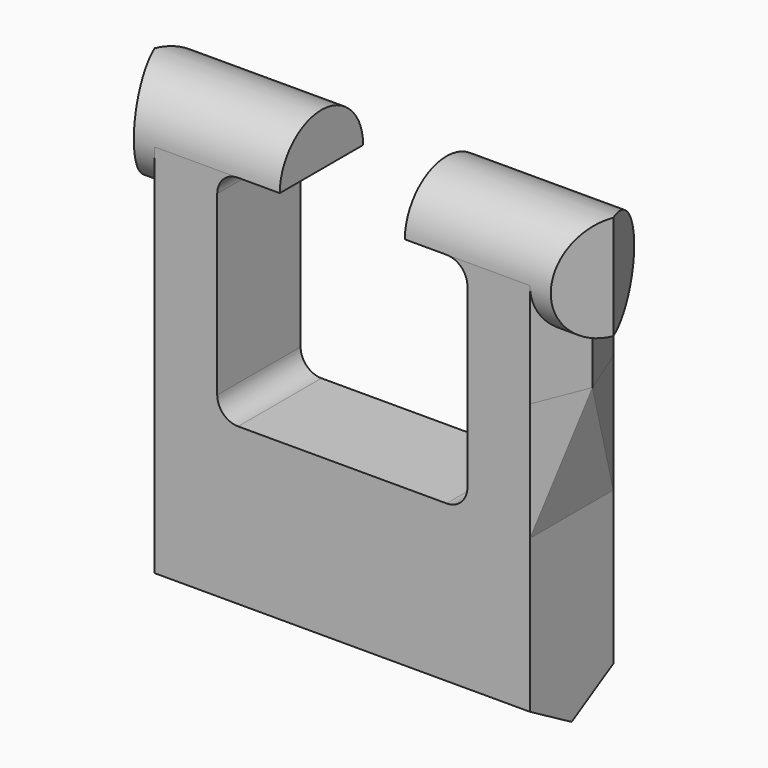
from build123d import *

# Parameters (mm, degrees)
F2_DEPTH     = 2.5
F3_DEPTH     = 10
F4_DEPTH     = 3
F5_DEPTH     = 6
F6_T1_DEPTH  = 5
F8_DEPTH     = 14
F9_DEPTH     = 9
F10_DEPTH    = 1
F11_DEPTH    = 16.5
F12_T4_DEPTH = 5
F14_DEPTH    = 6
F15_T1_DEPTH = 35.9238558823


# Not quite as in the source:
# - a fillet or chamfer that OpenCascade refuses, or shapes differently, is made with other operations: its cross-section is extruded or revolved along the edge and cut away or added


with BuildPart() as f2:
    # F0 (on Front) → F2 (new body, symmetric)
    with BuildSketch(Plane.XZ):
        Polygon((0, 3.5), (0, 0), (9, 0), (9, 14), (6, 14), (6, 3.5), align=None)
    extrude(amount=F2_DEPTH, both=True)

    # F1 (on Right) → F3 (join)
    with BuildSketch(Plane.YZ):
        with BuildLine():
            Line((-2.5, 14), (2.5, 14))
            ThreePointArc((2.5, 14), (0, 16.5), (-2.5, 14))
        make_face()
        with BuildLine():
            ThreePointArc((-2.5, 14), (0, 11.5), (2.5, 14))
            Line((2.5, 14), (-2.5, 14))
        make_face()
    extrude(amount=F3_DEPTH)

    # F1 (on Right) → F4 (cut)
    with BuildSketch(Plane.YZ):
        with BuildLine():
            Line((-2.5, 14), (2.5, 14))
            ThreePointArc((2.5, 14), (0, 16.5), (-2.5, 14))
        make_face()
        with BuildLine():
            ThreePointArc((-2.5, 14), (0, 11.5), (2.5, 14))
            Line((2.5, 14), (-2.5, 14))
        make_face()
    extrude(amount=F4_DEPTH, mode=Mode.SUBTRACT)

    # F1 (on Right) → F5 (cut)
    with BuildSketch(Plane.YZ):
        with BuildLine():
            ThreePointArc((-2.5, 14), (0, 11.5), (2.5, 14))
            Line((2.5, 14), (-2.5, 14))
        make_face()
    extrude(amount=F5_DEPTH, mode=Mode.SUBTRACT)

    # F6: fillet of radius 1 on 2 edges, made by hand

    # F6_s2 → F6_t1 (join)
    with BuildSketch(Plane.XZ.offset(-2.5)):
        with BuildLine():
            ThreePointArc((6, 13), (5.7071067812, 13.7071067812), (5, 14))
            Line((5, 14), (6, 14))
            Line((6, 14), (6, 13))
        make_face()
        with BuildLine():
            ThreePointArc((5, 3.5), (5.7071067812, 3.7928932188), (6, 4.5))
            Line((6, 4.5), (6, 3.5))
            Line((6, 3.5), (5, 3.5))
        make_face()
    extrude(amount=F6_T1_DEPTH)

    # F7 (on Top) → F8 (join)
    with BuildSketch(Plane.XY):
        Polygon((9, 2.5), (9, -2.5), (10, 0), align=None)
    extrude(amount=F8_DEPTH)

    # F7 (on Top) → F9 (cut)
    with BuildSketch(Plane.XY):
        Polygon((9, 2.5), (9, -2.5), (10, 0), align=None)
    extrude(amount=F9_DEPTH, mode=Mode.SUBTRACT)

    # F10 (add): a face of the model
    f10_faces = [f2.faces().sort_by_distance(p)[0] for p in [
        (10, -1.717766953, 12.282233047),
    ]]
    extrude(f10_faces, amount=F10_DEPTH)

    # F7 (on Top) → F11 (cut)
    with BuildSketch(Plane.XY):
        Polygon((11, 0), (10, -2.5), (11.5, -2.5), (11.5, 2.5), (10, 2.5), align=None)
    extrude(amount=F11_DEPTH, mode=Mode.SUBTRACT)

    # F12: chamfer of 1 x 5.6712818196 on 1 edges, made by hand


with BuildPart() as f12_tool2:
    # F12_s3 → F12_t4 (new body)
    with BuildSketch(Plane.XZ.offset(-2.5)):
        Polygon((10, 9), (9, 3.3287181804), (9, 9), align=None)
    extrude(amount=F12_T4_DEPTH)

    split(bisect_by=Plane(origin=(8.6206896552, 3.4482758621, 0), x_dir=(0, 0, 1), z_dir=(-0.9284766909, -0.3713906764, 0)), keep=Keep.TOP)

    split(bisect_by=Plane(origin=(8.6206896552, -3.4482758621, 0), x_dir=(0, 0, 1), z_dir=(-0.9284766909, 0.3713906764, 0)), keep=Keep.TOP)


with BuildPart() as f2_1:
    add(f2.part)

    # F12_t1: union F12_tool2
    add(f12_tool2.part)

    # F13: F2 across face


with BuildPart() as f2_2:
    add(f2_1.part)
    add(f2_1.part.mirror(Plane(origin=(0, 0, 1.75), x_dir=(0, -1, 0), z_dir=(-1, 0, 0))))

    # F14 (add): a face of the model
    f14_faces = [f2_2.faces().sort_by_distance(p)[0] for p in [
        (0, 0, 0),
    ]]
    extrude(f14_faces, amount=F14_DEPTH)

    # F15: chamfer of 2 x 3.4641016151 on 2 edges, made by hand

    # F15_s2 → F15_t1 (cut)
    with BuildSketch(Plane.YZ.offset(-17.9619279412)):
        Polygon((-2.5, -4), (0.9641016151, -6), (-2.5, -6), align=None)
        Polygon((-0.9641016151, -6), (2.5, -4), (2.5, -6), align=None)
    extrude(amount=F15_T1_DEPTH, mode=Mode.SUBTRACT)


solid = f2_2.part
